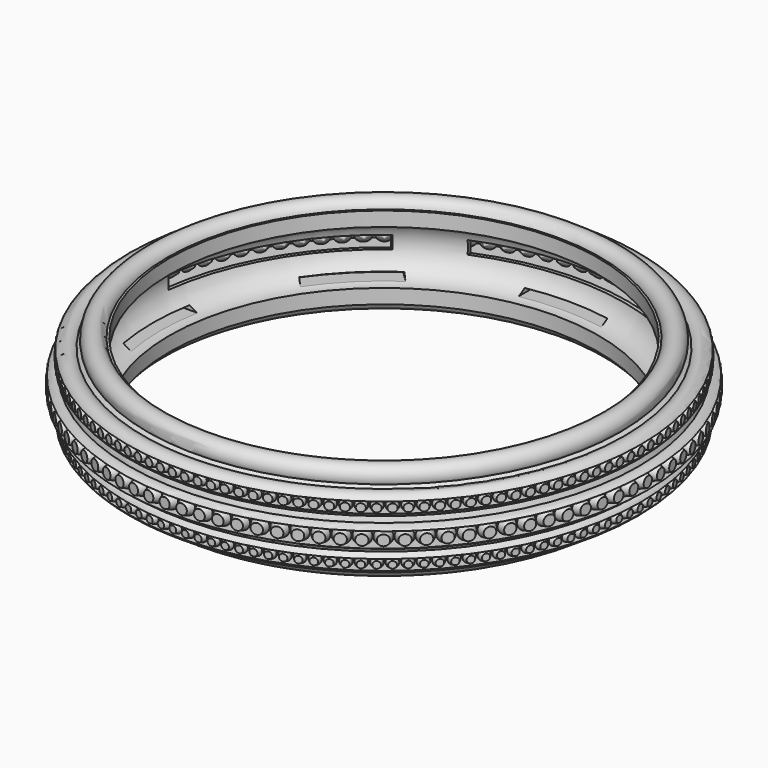
from build123d import *

# Parameters (mm, degrees)
F2_W      = 10.7606031051
F2_H      = 7.2111079935
F4_W      = 88.9
F4_H      = 6.096
F5_DEPTH  = 124.6271398151
F6_COUNT  = 6
F9_COUNT  = 98
F10_W     = 10.6947466134
F10_H     = 5.08
F10_W_2   = 9.758957445
F13_W     = 40.2778751929
F13_H     = 2.032
F13_W_2   = 39.1175959745
F14_DEPTH = 127
F15_COUNT = 8
F18_COUNT = 130
F21_COUNT = 130


with BuildPart() as f1:
    # F0 (on Front) → F1 (revolve)
    with BuildSketch(Plane.XZ):
        with BuildLine():
            ThreePointArc((101.6, 12.7), (114.3, 0), (101.6, -12.7))
            Line((101.6, -12.7), (101.6, -19.5476406297))
            ThreePointArc((101.6, -19.5476406297), (102.0112979939, -19.5433131313), (102.4224138798, -19.5303325521))
            ThreePointArc((102.4224138798, -19.5303325521), (108.4539940671, -23.3155491771), (111.4776025264, -16.8684090096))
            ThreePointArc((111.4776025264, -16.8684090096), (112.6214083664, -16.1443120574), (113.712355318, -15.3427866712))
            ThreePointArc((113.712355318, -15.3427866712), (121.1960862403, -14.7794979456), (119.6808746024, -7.4291471785))
            ThreePointArc((119.6808746024, -7.4291471785), (120.1341217826, -6.2126149032), (120.5056200226, -4.9686804834))
            ThreePointArc((120.5056200226, -4.9686804834), (126.157628275, 0), (120.5056200226, 4.9686804834))
            ThreePointArc((120.5056200226, 4.9686804834), (120.141776973, 6.1897302745), (119.6991616614, 7.3844838236))
            ThreePointArc((119.6991616614, 7.3844838236), (121.234298908, 14.8083181925), (113.674437882, 15.3726446658))
            ThreePointArc((113.674437882, 15.3726446658), (112.8348855677, 15.996487129), (111.963166428, 16.5745297301))
            ThreePointArc((111.963166428, 16.5745297301), (108.9586357212, 23.360226878), (102.6073888593, 19.5216654482))
            ThreePointArc((102.6073888593, 19.5216654482), (102.1038618421, 19.5411457553), (101.6, 19.5476406297))
            Line((101.6, 19.5476406297), (101.6, 12.7))
        make_face()
    revolve(axis=Axis((0, 0, 0.8939662948), (0, 0, -1)))

    # F2 (on Front) → F3 (revolve, cut)
    with BuildSketch(Plane.XZ):
        with Locations((121.0180819035, 0)):
            Rectangle(F2_W, F2_H)
    revolve(axis=Axis((0, 0, 0.6015782217), (0, 0, -1)), mode=Mode.SUBTRACT)

    # F4 (on Front) → F5 (cut, through all)
    with BuildSketch(Plane.XZ):
        Rectangle(F4_W, F4_H)
    f5 = extrude(amount=F5_DEPTH, mode=Mode.SUBTRACT)

    # F6: F5 ×6 about axis
    f6_axis = Axis((0, 0, 0.6015782217), (0, 0, -1))
    for i in range(1, F6_COUNT):
        add(f5.rotate(f6_axis, i * 360 / F6_COUNT), mode=Mode.SUBTRACT)

    # F10 (on Front) → F12 (revolve, cut)
    with BuildSketch(Plane.XZ):
        with Locations((118.0006936193, 11.8413660675)):
            Rectangle(F10_W, F10_H)
        with Locations((118.0006936193, -12.040737085)):
            Rectangle(F10_W_2, F10_H)
    revolve(axis=Axis((0, 0, 3.7605240941), (0, 0, -1)), mode=Mode.SUBTRACT)

    # F13 (on Front) → F14 (cut)
    with BuildSketch(Plane.XZ):
        with Locations((0, 10.9197665006)):
            Rectangle(F13_W, F13_H)
        with Locations((0, -10.9790544957)):
            Rectangle(F13_W_2, F13_H)
    f14 = extrude(amount=F14_DEPTH, mode=Mode.SUBTRACT)

    # F15: F14 ×8 about axis
    f15_axis = Axis((0, 0, 3.7605240941), (0, 0, -1))
    for i in range(1, F15_COUNT):
        add(f14.rotate(f15_axis, i * 360 / F15_COUNT), mode=Mode.SUBTRACT)


with BuildPart() as f8:
    # F7 (on Front) → F8 (revolve)
    with BuildSketch(Plane.XZ):
        Polygon((121.5662360191, 3.7640826777), (117.0876398683, 0), (124.899148941, 0), (124.899148941, 2.4697111055), align=None)
    revolve(axis=Axis((124.899148941, 0, 0), (1, 0, 0)))


with BuildPart() as f9_1:
    # F9: instance of F8
    add(f8.part.rotate(Axis((0, 0, 0.6015782217), (0, 0, -1)), 1 * 360 / F9_COUNT))


with BuildPart() as f9_2:
    # F9: instance of F8
    add(f8.part.rotate(Axis((0, 0, 0.6015782217), (0, 0, -1)), 2 * 360 / F9_COUNT))


with BuildPart() as f9_3:
    # F9: instance of F8
    add(f8.part.rotate(Axis((0, 0, 0.6015782217), (0, 0, -1)), 3 * 360 / F9_COUNT))


with BuildPart() as f9_4:
    # F9: instance of F8
    add(f8.part.rotate(Axis((0, 0, 0.6015782217), (0, 0, -1)), 4 * 360 / F9_COUNT))


with BuildPart() as f9_5:
    # F9: instance of F8
    add(f8.part.rotate(Axis((0, 0, 0.6015782217), (0, 0, -1)), 5 * 360 / F9_COUNT))


with BuildPart() as f9_6:
    # F9: instance of F8
    add(f8.part.rotate(Axis((0, 0, 0.6015782217), (0, 0, -1)), 6 * 360 / F9_COUNT))


with BuildPart() as f9_7:
    # F9: instance of F8
    add(f8.part.rotate(Axis((0, 0, 0.6015782217), (0, 0, -1)), 7 * 360 / F9_COUNT))


with BuildPart() as f9_8:
    # F9: instance of F8
    add(f8.part.rotate(Axis((0, 0, 0.6015782217), (0, 0, -1)), 8 * 360 / F9_COUNT))


with BuildPart() as f9_9:
    # F9: instance of F8
    add(f8.part.rotate(Axis((0, 0, 0.6015782217), (0, 0, -1)), 9 * 360 / F9_COUNT))


with BuildPart() as f9_10:
    # F9: instance of F8
    add(f8.part.rotate(Axis((0, 0, 0.6015782217), (0, 0, -1)), 10 * 360 / F9_COUNT))


with BuildPart() as f9_11:
    # F9: instance of F8
    add(f8.part.rotate(Axis((0, 0, 0.6015782217), (0, 0, -1)), 11 * 360 / F9_COUNT))


with BuildPart() as f9_12:
    # F9: instance of F8
    add(f8.part.rotate(Axis((0, 0, 0.6015782217), (0, 0, -1)), 12 * 360 / F9_COUNT))


with BuildPart() as f9_13:
    # F9: instance of F8
    add(f8.part.rotate(Axis((0, 0, 0.6015782217), (0, 0, -1)), 13 * 360 / F9_COUNT))


with BuildPart() as f9_14:
    # F9: instance of F8
    add(f8.part.rotate(Axis((0, 0, 0.6015782217), (0, 0, -1)), 14 * 360 / F9_COUNT))


with BuildPart() as f9_15:
    # F9: instance of F8
    add(f8.part.rotate(Axis((0, 0, 0.6015782217), (0, 0, -1)), 15 * 360 / F9_COUNT))


with BuildPart() as f9_16:
    # F9: instance of F8
    add(f8.part.rotate(Axis((0, 0, 0.6015782217), (0, 0, -1)), 16 * 360 / F9_COUNT))


with BuildPart() as f9_17:
    # F9: instance of F8
    add(f8.part.rotate(Axis((0, 0, 0.6015782217), (0, 0, -1)), 17 * 360 / F9_COUNT))


with BuildPart() as f9_18:
    # F9: instance of F8
    add(f8.part.rotate(Axis((0, 0, 0.6015782217), (0, 0, -1)), 18 * 360 / F9_COUNT))


with BuildPart() as f9_19:
    # F9: instance of F8
    add(f8.part.rotate(Axis((0, 0, 0.6015782217), (0, 0, -1)), 19 * 360 / F9_COUNT))


with BuildPart() as f9_20:
    # F9: instance of F8
    add(f8.part.rotate(Axis((0, 0, 0.6015782217), (0, 0, -1)), 20 * 360 / F9_COUNT))


with BuildPart() as f9_21:
    # F9: instance of F8
    add(f8.part.rotate(Axis((0, 0, 0.6015782217), (0, 0, -1)), 21 * 360 / F9_COUNT))


with BuildPart() as f9_22:
    # F9: instance of F8
    add(f8.part.rotate(Axis((0, 0, 0.6015782217), (0, 0, -1)), 22 * 360 / F9_COUNT))


with BuildPart() as f9_23:
    # F9: instance of F8
    add(f8.part.rotate(Axis((0, 0, 0.6015782217), (0, 0, -1)), 23 * 360 / F9_COUNT))


with BuildPart() as f9_24:
    # F9: instance of F8
    add(f8.part.rotate(Axis((0, 0, 0.6015782217), (0, 0, -1)), 24 * 360 / F9_COUNT))


with BuildPart() as f9_25:
    # F9: instance of F8
    add(f8.part.rotate(Axis((0, 0, 0.6015782217), (0, 0, -1)), 25 * 360 / F9_COUNT))


with BuildPart() as f9_26:
    # F9: instance of F8
    add(f8.part.rotate(Axis((0, 0, 0.6015782217), (0, 0, -1)), 26 * 360 / F9_COUNT))


with BuildPart() as f9_27:
    # F9: instance of F8
    add(f8.part.rotate(Axis((0, 0, 0.6015782217), (0, 0, -1)), 27 * 360 / F9_COUNT))


with BuildPart() as f9_28:
    # F9: instance of F8
    add(f8.part.rotate(Axis((0, 0, 0.6015782217), (0, 0, -1)), 28 * 360 / F9_COUNT))


with BuildPart() as f9_29:
    # F9: instance of F8
    add(f8.part.rotate(Axis((0, 0, 0.6015782217), (0, 0, -1)), 29 * 360 / F9_COUNT))


with BuildPart() as f9_30:
    # F9: instance of F8
    add(f8.part.rotate(Axis((0, 0, 0.6015782217), (0, 0, -1)), 30 * 360 / F9_COUNT))


with BuildPart() as f9_31:
    # F9: instance of F8
    add(f8.part.rotate(Axis((0, 0, 0.6015782217), (0, 0, -1)), 31 * 360 / F9_COUNT))


with BuildPart() as f9_32:
    # F9: instance of F8
    add(f8.part.rotate(Axis((0, 0, 0.6015782217), (0, 0, -1)), 32 * 360 / F9_COUNT))


with BuildPart() as f9_33:
    # F9: instance of F8
    add(f8.part.rotate(Axis((0, 0, 0.6015782217), (0, 0, -1)), 33 * 360 / F9_COUNT))


with BuildPart() as f9_34:
    # F9: instance of F8
    add(f8.part.rotate(Axis((0, 0, 0.6015782217), (0, 0, -1)), 34 * 360 / F9_COUNT))


with BuildPart() as f9_35:
    # F9: instance of F8
    add(f8.part.rotate(Axis((0, 0, 0.6015782217), (0, 0, -1)), 35 * 360 / F9_COUNT))


with BuildPart() as f9_36:
    # F9: instance of F8
    add(f8.part.rotate(Axis((0, 0, 0.6015782217), (0, 0, -1)), 36 * 360 / F9_COUNT))


with BuildPart() as f9_37:
    # F9: instance of F8
    add(f8.part.rotate(Axis((0, 0, 0.6015782217), (0, 0, -1)), 37 * 360 / F9_COUNT))


with BuildPart() as f9_38:
    # F9: instance of F8
    add(f8.part.rotate(Axis((0, 0, 0.6015782217), (0, 0, -1)), 38 * 360 / F9_COUNT))


with BuildPart() as f9_39:
    # F9: instance of F8
    add(f8.part.rotate(Axis((0, 0, 0.6015782217), (0, 0, -1)), 39 * 360 / F9_COUNT))


with BuildPart() as f9_40:
    # F9: instance of F8
    add(f8.part.rotate(Axis((0, 0, 0.6015782217), (0, 0, -1)), 40 * 360 / F9_COUNT))


with BuildPart() as f9_41:
    # F9: instance of F8
    add(f8.part.rotate(Axis((0, 0, 0.6015782217), (0, 0, -1)), 41 * 360 / F9_COUNT))


with BuildPart() as f9_42:
    # F9: instance of F8
    add(f8.part.rotate(Axis((0, 0, 0.6015782217), (0, 0, -1)), 42 * 360 / F9_COUNT))


with BuildPart() as f9_43:
    # F9: instance of F8
    add(f8.part.rotate(Axis((0, 0, 0.6015782217), (0, 0, -1)), 43 * 360 / F9_COUNT))


with BuildPart() as f9_44:
    # F9: instance of F8
    add(f8.part.rotate(Axis((0, 0, 0.6015782217), (0, 0, -1)), 44 * 360 / F9_COUNT))


with BuildPart() as f9_45:
    # F9: instance of F8
    add(f8.part.rotate(Axis((0, 0, 0.6015782217), (0, 0, -1)), 45 * 360 / F9_COUNT))


with BuildPart() as f9_46:
    # F9: instance of F8
    add(f8.part.rotate(Axis((0, 0, 0.6015782217), (0, 0, -1)), 46 * 360 / F9_COUNT))


with BuildPart() as f9_47:
    # F9: instance of F8
    add(f8.part.rotate(Axis((0, 0, 0.6015782217), (0, 0, -1)), 47 * 360 / F9_COUNT))


with BuildPart() as f9_48:
    # F9: instance of F8
    add(f8.part.rotate(Axis((0, 0, 0.6015782217), (0, 0, -1)), 48 * 360 / F9_COUNT))


with BuildPart() as f9_49:
    # F9: instance of F8
    add(f8.part.rotate(Axis((0, 0, 0.6015782217), (0, 0, -1)), 49 * 360 / F9_COUNT))


with BuildPart() as f9_50:
    # F9: instance of F8
    add(f8.part.rotate(Axis((0, 0, 0.6015782217), (0, 0, -1)), 50 * 360 / F9_COUNT))


with BuildPart() as f9_51:
    # F9: instance of F8
    add(f8.part.rotate(Axis((0, 0, 0.6015782217), (0, 0, -1)), 51 * 360 / F9_COUNT))


with BuildPart() as f9_52:
    # F9: instance of F8
    add(f8.part.rotate(Axis((0, 0, 0.6015782217), (0, 0, -1)), 52 * 360 / F9_COUNT))


with BuildPart() as f9_53:
    # F9: instance of F8
    add(f8.part.rotate(Axis((0, 0, 0.6015782217), (0, 0, -1)), 53 * 360 / F9_COUNT))


with BuildPart() as f9_54:
    # F9: instance of F8
    add(f8.part.rotate(Axis((0, 0, 0.6015782217), (0, 0, -1)), 54 * 360 / F9_COUNT))


with BuildPart() as f9_55:
    # F9: instance of F8
    add(f8.part.rotate(Axis((0, 0, 0.6015782217), (0, 0, -1)), 55 * 360 / F9_COUNT))


with BuildPart() as f9_56:
    # F9: instance of F8
    add(f8.part.rotate(Axis((0, 0, 0.6015782217), (0, 0, -1)), 56 * 360 / F9_COUNT))


with BuildPart() as f9_57:
    # F9: instance of F8
    add(f8.part.rotate(Axis((0, 0, 0.6015782217), (0, 0, -1)), 57 * 360 / F9_COUNT))


with BuildPart() as f9_58:
    # F9: instance of F8
    add(f8.part.rotate(Axis((0, 0, 0.6015782217), (0, 0, -1)), 58 * 360 / F9_COUNT))


with BuildPart() as f9_59:
    # F9: instance of F8
    add(f8.part.rotate(Axis((0, 0, 0.6015782217), (0, 0, -1)), 59 * 360 / F9_COUNT))


with BuildPart() as f9_60:
    # F9: instance of F8
    add(f8.part.rotate(Axis((0, 0, 0.6015782217), (0, 0, -1)), 60 * 360 / F9_COUNT))


with BuildPart() as f9_61:
    # F9: instance of F8
    add(f8.part.rotate(Axis((0, 0, 0.6015782217), (0, 0, -1)), 61 * 360 / F9_COUNT))


with BuildPart() as f9_62:
    # F9: instance of F8
    add(f8.part.rotate(Axis((0, 0, 0.6015782217), (0, 0, -1)), 62 * 360 / F9_COUNT))


with BuildPart() as f9_63:
    # F9: instance of F8
    add(f8.part.rotate(Axis((0, 0, 0.6015782217), (0, 0, -1)), 63 * 360 / F9_COUNT))


with BuildPart() as f9_64:
    # F9: instance of F8
    add(f8.part.rotate(Axis((0, 0, 0.6015782217), (0, 0, -1)), 64 * 360 / F9_COUNT))


with BuildPart() as f9_65:
    # F9: instance of F8
    add(f8.part.rotate(Axis((0, 0, 0.6015782217), (0, 0, -1)), 65 * 360 / F9_COUNT))


with BuildPart() as f9_66:
    # F9: instance of F8
    add(f8.part.rotate(Axis((0, 0, 0.6015782217), (0, 0, -1)), 66 * 360 / F9_COUNT))


with BuildPart() as f9_67:
    # F9: instance of F8
    add(f8.part.rotate(Axis((0, 0, 0.6015782217), (0, 0, -1)), 67 * 360 / F9_COUNT))


with BuildPart() as f9_68:
    # F9: instance of F8
    add(f8.part.rotate(Axis((0, 0, 0.6015782217), (0, 0, -1)), 68 * 360 / F9_COUNT))


with BuildPart() as f9_69:
    # F9: instance of F8
    add(f8.part.rotate(Axis((0, 0, 0.6015782217), (0, 0, -1)), 69 * 360 / F9_COUNT))


with BuildPart() as f9_70:
    # F9: instance of F8
    add(f8.part.rotate(Axis((0, 0, 0.6015782217), (0, 0, -1)), 70 * 360 / F9_COUNT))


with BuildPart() as f9_71:
    # F9: instance of F8
    add(f8.part.rotate(Axis((0, 0, 0.6015782217), (0, 0, -1)), 71 * 360 / F9_COUNT))


with BuildPart() as f9_72:
    # F9: instance of F8
    add(f8.part.rotate(Axis((0, 0, 0.6015782217), (0, 0, -1)), 72 * 360 / F9_COUNT))


with BuildPart() as f9_73:
    # F9: instance of F8
    add(f8.part.rotate(Axis((0, 0, 0.6015782217), (0, 0, -1)), 73 * 360 / F9_COUNT))


with BuildPart() as f9_74:
    # F9: instance of F8
    add(f8.part.rotate(Axis((0, 0, 0.6015782217), (0, 0, -1)), 74 * 360 / F9_COUNT))


with BuildPart() as f9_75:
    # F9: instance of F8
    add(f8.part.rotate(Axis((0, 0, 0.6015782217), (0, 0, -1)), 75 * 360 / F9_COUNT))


with BuildPart() as f9_76:
    # F9: instance of F8
    add(f8.part.rotate(Axis((0, 0, 0.6015782217), (0, 0, -1)), 76 * 360 / F9_COUNT))


with BuildPart() as f9_77:
    # F9: instance of F8
    add(f8.part.rotate(Axis((0, 0, 0.6015782217), (0, 0, -1)), 77 * 360 / F9_COUNT))


with BuildPart() as f9_78:
    # F9: instance of F8
    add(f8.part.rotate(Axis((0, 0, 0.6015782217), (0, 0, -1)), 78 * 360 / F9_COUNT))


with BuildPart() as f9_79:
    # F9: instance of F8
    add(f8.part.rotate(Axis((0, 0, 0.6015782217), (0, 0, -1)), 79 * 360 / F9_COUNT))


with BuildPart() as f9_80:
    # F9: instance of F8
    add(f8.part.rotate(Axis((0, 0, 0.6015782217), (0, 0, -1)), 80 * 360 / F9_COUNT))


with BuildPart() as f9_81:
    # F9: instance of F8
    add(f8.part.rotate(Axis((0, 0, 0.6015782217), (0, 0, -1)), 81 * 360 / F9_COUNT))


with BuildPart() as f9_82:
    # F9: instance of F8
    add(f8.part.rotate(Axis((0, 0, 0.6015782217), (0, 0, -1)), 82 * 360 / F9_COUNT))


with BuildPart() as f9_83:
    # F9: instance of F8
    add(f8.part.rotate(Axis((0, 0, 0.6015782217), (0, 0, -1)), 83 * 360 / F9_COUNT))


with BuildPart() as f9_84:
    # F9: instance of F8
    add(f8.part.rotate(Axis((0, 0, 0.6015782217), (0, 0, -1)), 84 * 360 / F9_COUNT))


with BuildPart() as f9_85:
    # F9: instance of F8
    add(f8.part.rotate(Axis((0, 0, 0.6015782217), (0, 0, -1)), 85 * 360 / F9_COUNT))


with BuildPart() as f9_86:
    # F9: instance of F8
    add(f8.part.rotate(Axis((0, 0, 0.6015782217), (0, 0, -1)), 86 * 360 / F9_COUNT))


with BuildPart() as f9_87:
    # F9: instance of F8
    add(f8.part.rotate(Axis((0, 0, 0.6015782217), (0, 0, -1)), 87 * 360 / F9_COUNT))


with BuildPart() as f9_88:
    # F9: instance of F8
    add(f8.part.rotate(Axis((0, 0, 0.6015782217), (0, 0, -1)), 88 * 360 / F9_COUNT))


with BuildPart() as f9_89:
    # F9: instance of F8
    add(f8.part.rotate(Axis((0, 0, 0.6015782217), (0, 0, -1)), 89 * 360 / F9_COUNT))


with BuildPart() as f9_90:
    # F9: instance of F8
    add(f8.part.rotate(Axis((0, 0, 0.6015782217), (0, 0, -1)), 90 * 360 / F9_COUNT))


with BuildPart() as f9_91:
    # F9: instance of F8
    add(f8.part.rotate(Axis((0, 0, 0.6015782217), (0, 0, -1)), 91 * 360 / F9_COUNT))


with BuildPart() as f9_92:
    # F9: instance of F8
    add(f8.part.rotate(Axis((0, 0, 0.6015782217), (0, 0, -1)), 92 * 360 / F9_COUNT))


with BuildPart() as f9_93:
    # F9: instance of F8
    add(f8.part.rotate(Axis((0, 0, 0.6015782217), (0, 0, -1)), 93 * 360 / F9_COUNT))


with BuildPart() as f9_94:
    # F9: instance of F8
    add(f8.part.rotate(Axis((0, 0, 0.6015782217), (0, 0, -1)), 94 * 360 / F9_COUNT))


with BuildPart() as f9_95:
    # F9: instance of F8
    add(f8.part.rotate(Axis((0, 0, 0.6015782217), (0, 0, -1)), 95 * 360 / F9_COUNT))


with BuildPart() as f9_96:
    # F9: instance of F8
    add(f8.part.rotate(Axis((0, 0, 0.6015782217), (0, 0, -1)), 96 * 360 / F9_COUNT))


with BuildPart() as f9_97:
    # F9: instance of F8
    add(f8.part.rotate(Axis((0, 0, 0.6015782217), (0, 0, -1)), 97 * 360 / F9_COUNT))


with BuildPart() as f17:
    # F16 (on Front) → F17 (revolve)
    with BuildSketch(Plane.XZ):
        Polygon((115.7522408575, 11.8132652715), (121.7399388552, 11.8132652715), (121.7399388552, 13.6975445746), (119.4161549211, 14.4187174737), align=None)
    revolve(axis=Axis((116.3177825511, 0, 11.8132652715), (1, 0, 0)))


with BuildPart() as f18_1:
    # F18: instance of F17
    add(f17.part.rotate(Axis((0, 0, 3.7605240941), (0, 0, -1)), 1 * 360 / F18_COUNT))


with BuildPart() as f18_2:
    # F18: instance of F17
    add(f17.part.rotate(Axis((0, 0, 3.7605240941), (0, 0, -1)), 2 * 360 / F18_COUNT))


with BuildPart() as f18_3:
    # F18: instance of F17
    add(f17.part.rotate(Axis((0, 0, 3.7605240941), (0, 0, -1)), 3 * 360 / F18_COUNT))


with BuildPart() as f18_4:
    # F18: instance of F17
    add(f17.part.rotate(Axis((0, 0, 3.7605240941), (0, 0, -1)), 4 * 360 / F18_COUNT))


with BuildPart() as f18_5:
    # F18: instance of F17
    add(f17.part.rotate(Axis((0, 0, 3.7605240941), (0, 0, -1)), 5 * 360 / F18_COUNT))


with BuildPart() as f18_6:
    # F18: instance of F17
    add(f17.part.rotate(Axis((0, 0, 3.7605240941), (0, 0, -1)), 6 * 360 / F18_COUNT))


with BuildPart() as f18_7:
    # F18: instance of F17
    add(f17.part.rotate(Axis((0, 0, 3.7605240941), (0, 0, -1)), 7 * 360 / F18_COUNT))


with BuildPart() as f18_8:
    # F18: instance of F17
    add(f17.part.rotate(Axis((0, 0, 3.7605240941), (0, 0, -1)), 8 * 360 / F18_COUNT))


with BuildPart() as f18_9:
    # F18: instance of F17
    add(f17.part.rotate(Axis((0, 0, 3.7605240941), (0, 0, -1)), 9 * 360 / F18_COUNT))


with BuildPart() as f18_10:
    # F18: instance of F17
    add(f17.part.rotate(Axis((0, 0, 3.7605240941), (0, 0, -1)), 10 * 360 / F18_COUNT))


with BuildPart() as f18_11:
    # F18: instance of F17
    add(f17.part.rotate(Axis((0, 0, 3.7605240941), (0, 0, -1)), 11 * 360 / F18_COUNT))


with BuildPart() as f18_12:
    # F18: instance of F17
    add(f17.part.rotate(Axis((0, 0, 3.7605240941), (0, 0, -1)), 12 * 360 / F18_COUNT))


with BuildPart() as f18_13:
    # F18: instance of F17
    add(f17.part.rotate(Axis((0, 0, 3.7605240941), (0, 0, -1)), 13 * 360 / F18_COUNT))


with BuildPart() as f18_14:
    # F18: instance of F17
    add(f17.part.rotate(Axis((0, 0, 3.7605240941), (0, 0, -1)), 14 * 360 / F18_COUNT))


with BuildPart() as f18_15:
    # F18: instance of F17
    add(f17.part.rotate(Axis((0, 0, 3.7605240941), (0, 0, -1)), 15 * 360 / F18_COUNT))


with BuildPart() as f18_16:
    # F18: instance of F17
    add(f17.part.rotate(Axis((0, 0, 3.7605240941), (0, 0, -1)), 16 * 360 / F18_COUNT))


with BuildPart() as f18_17:
    # F18: instance of F17
    add(f17.part.rotate(Axis((0, 0, 3.7605240941), (0, 0, -1)), 17 * 360 / F18_COUNT))


with BuildPart() as f18_18:
    # F18: instance of F17
    add(f17.part.rotate(Axis((0, 0, 3.7605240941), (0, 0, -1)), 18 * 360 / F18_COUNT))


with BuildPart() as f18_19:
    # F18: instance of F17
    add(f17.part.rotate(Axis((0, 0, 3.7605240941), (0, 0, -1)), 19 * 360 / F18_COUNT))


with BuildPart() as f18_20:
    # F18: instance of F17
    add(f17.part.rotate(Axis((0, 0, 3.7605240941), (0, 0, -1)), 20 * 360 / F18_COUNT))


with BuildPart() as f18_21:
    # F18: instance of F17
    add(f17.part.rotate(Axis((0, 0, 3.7605240941), (0, 0, -1)), 21 * 360 / F18_COUNT))


with BuildPart() as f18_22:
    # F18: instance of F17
    add(f17.part.rotate(Axis((0, 0, 3.7605240941), (0, 0, -1)), 22 * 360 / F18_COUNT))


with BuildPart() as f18_23:
    # F18: instance of F17
    add(f17.part.rotate(Axis((0, 0, 3.7605240941), (0, 0, -1)), 23 * 360 / F18_COUNT))


with BuildPart() as f18_24:
    # F18: instance of F17
    add(f17.part.rotate(Axis((0, 0, 3.7605240941), (0, 0, -1)), 24 * 360 / F18_COUNT))


with BuildPart() as f18_25:
    # F18: instance of F17
    add(f17.part.rotate(Axis((0, 0, 3.7605240941), (0, 0, -1)), 25 * 360 / F18_COUNT))


with BuildPart() as f18_26:
    # F18: instance of F17
    add(f17.part.rotate(Axis((0, 0, 3.7605240941), (0, 0, -1)), 26 * 360 / F18_COUNT))


with BuildPart() as f18_27:
    # F18: instance of F17
    add(f17.part.rotate(Axis((0, 0, 3.7605240941), (0, 0, -1)), 27 * 360 / F18_COUNT))


with BuildPart() as f18_28:
    # F18: instance of F17
    add(f17.part.rotate(Axis((0, 0, 3.7605240941), (0, 0, -1)), 28 * 360 / F18_COUNT))


with BuildPart() as f18_29:
    # F18: instance of F17
    add(f17.part.rotate(Axis((0, 0, 3.7605240941), (0, 0, -1)), 29 * 360 / F18_COUNT))


with BuildPart() as f18_30:
    # F18: instance of F17
    add(f17.part.rotate(Axis((0, 0, 3.7605240941), (0, 0, -1)), 30 * 360 / F18_COUNT))


with BuildPart() as f18_31:
    # F18: instance of F17
    add(f17.part.rotate(Axis((0, 0, 3.7605240941), (0, 0, -1)), 31 * 360 / F18_COUNT))


with BuildPart() as f18_32:
    # F18: instance of F17
    add(f17.part.rotate(Axis((0, 0, 3.7605240941), (0, 0, -1)), 32 * 360 / F18_COUNT))


with BuildPart() as f18_33:
    # F18: instance of F17
    add(f17.part.rotate(Axis((0, 0, 3.7605240941), (0, 0, -1)), 33 * 360 / F18_COUNT))


with BuildPart() as f18_34:
    # F18: instance of F17
    add(f17.part.rotate(Axis((0, 0, 3.7605240941), (0, 0, -1)), 34 * 360 / F18_COUNT))


with BuildPart() as f18_35:
    # F18: instance of F17
    add(f17.part.rotate(Axis((0, 0, 3.7605240941), (0, 0, -1)), 35 * 360 / F18_COUNT))


with BuildPart() as f18_36:
    # F18: instance of F17
    add(f17.part.rotate(Axis((0, 0, 3.7605240941), (0, 0, -1)), 36 * 360 / F18_COUNT))


with BuildPart() as f18_37:
    # F18: instance of F17
    add(f17.part.rotate(Axis((0, 0, 3.7605240941), (0, 0, -1)), 37 * 360 / F18_COUNT))


with BuildPart() as f18_38:
    # F18: instance of F17
    add(f17.part.rotate(Axis((0, 0, 3.7605240941), (0, 0, -1)), 38 * 360 / F18_COUNT))


with BuildPart() as f18_39:
    # F18: instance of F17
    add(f17.part.rotate(Axis((0, 0, 3.7605240941), (0, 0, -1)), 39 * 360 / F18_COUNT))


with BuildPart() as f18_40:
    # F18: instance of F17
    add(f17.part.rotate(Axis((0, 0, 3.7605240941), (0, 0, -1)), 40 * 360 / F18_COUNT))


with BuildPart() as f18_41:
    # F18: instance of F17
    add(f17.part.rotate(Axis((0, 0, 3.7605240941), (0, 0, -1)), 41 * 360 / F18_COUNT))


with BuildPart() as f18_42:
    # F18: instance of F17
    add(f17.part.rotate(Axis((0, 0, 3.7605240941), (0, 0, -1)), 42 * 360 / F18_COUNT))


with BuildPart() as f18_43:
    # F18: instance of F17
    add(f17.part.rotate(Axis((0, 0, 3.7605240941), (0, 0, -1)), 43 * 360 / F18_COUNT))


with BuildPart() as f18_44:
    # F18: instance of F17
    add(f17.part.rotate(Axis((0, 0, 3.7605240941), (0, 0, -1)), 44 * 360 / F18_COUNT))


with BuildPart() as f18_45:
    # F18: instance of F17
    add(f17.part.rotate(Axis((0, 0, 3.7605240941), (0, 0, -1)), 45 * 360 / F18_COUNT))


with BuildPart() as f18_46:
    # F18: instance of F17
    add(f17.part.rotate(Axis((0, 0, 3.7605240941), (0, 0, -1)), 46 * 360 / F18_COUNT))


with BuildPart() as f18_47:
    # F18: instance of F17
    add(f17.part.rotate(Axis((0, 0, 3.7605240941), (0, 0, -1)), 47 * 360 / F18_COUNT))


with BuildPart() as f18_48:
    # F18: instance of F17
    add(f17.part.rotate(Axis((0, 0, 3.7605240941), (0, 0, -1)), 48 * 360 / F18_COUNT))


with BuildPart() as f18_49:
    # F18: instance of F17
    add(f17.part.rotate(Axis((0, 0, 3.7605240941), (0, 0, -1)), 49 * 360 / F18_COUNT))


with BuildPart() as f18_50:
    # F18: instance of F17
    add(f17.part.rotate(Axis((0, 0, 3.7605240941), (0, 0, -1)), 50 * 360 / F18_COUNT))


with BuildPart() as f18_51:
    # F18: instance of F17
    add(f17.part.rotate(Axis((0, 0, 3.7605240941), (0, 0, -1)), 51 * 360 / F18_COUNT))


with BuildPart() as f18_52:
    # F18: instance of F17
    add(f17.part.rotate(Axis((0, 0, 3.7605240941), (0, 0, -1)), 52 * 360 / F18_COUNT))


with BuildPart() as f18_53:
    # F18: instance of F17
    add(f17.part.rotate(Axis((0, 0, 3.7605240941), (0, 0, -1)), 53 * 360 / F18_COUNT))


with BuildPart() as f18_54:
    # F18: instance of F17
    add(f17.part.rotate(Axis((0, 0, 3.7605240941), (0, 0, -1)), 54 * 360 / F18_COUNT))


with BuildPart() as f18_55:
    # F18: instance of F17
    add(f17.part.rotate(Axis((0, 0, 3.7605240941), (0, 0, -1)), 55 * 360 / F18_COUNT))


with BuildPart() as f18_56:
    # F18: instance of F17
    add(f17.part.rotate(Axis((0, 0, 3.7605240941), (0, 0, -1)), 56 * 360 / F18_COUNT))


with BuildPart() as f18_57:
    # F18: instance of F17
    add(f17.part.rotate(Axis((0, 0, 3.7605240941), (0, 0, -1)), 57 * 360 / F18_COUNT))


with BuildPart() as f18_58:
    # F18: instance of F17
    add(f17.part.rotate(Axis((0, 0, 3.7605240941), (0, 0, -1)), 58 * 360 / F18_COUNT))


with BuildPart() as f18_59:
    # F18: instance of F17
    add(f17.part.rotate(Axis((0, 0, 3.7605240941), (0, 0, -1)), 59 * 360 / F18_COUNT))


with BuildPart() as f18_60:
    # F18: instance of F17
    add(f17.part.rotate(Axis((0, 0, 3.7605240941), (0, 0, -1)), 60 * 360 / F18_COUNT))


with BuildPart() as f18_61:
    # F18: instance of F17
    add(f17.part.rotate(Axis((0, 0, 3.7605240941), (0, 0, -1)), 61 * 360 / F18_COUNT))


with BuildPart() as f18_62:
    # F18: instance of F17
    add(f17.part.rotate(Axis((0, 0, 3.7605240941), (0, 0, -1)), 62 * 360 / F18_COUNT))


with BuildPart() as f18_63:
    # F18: instance of F17
    add(f17.part.rotate(Axis((0, 0, 3.7605240941), (0, 0, -1)), 63 * 360 / F18_COUNT))


with BuildPart() as f18_64:
    # F18: instance of F17
    add(f17.part.rotate(Axis((0, 0, 3.7605240941), (0, 0, -1)), 64 * 360 / F18_COUNT))


with BuildPart() as f18_65:
    # F18: instance of F17
    add(f17.part.rotate(Axis((0, 0, 3.7605240941), (0, 0, -1)), 65 * 360 / F18_COUNT))


with BuildPart() as f18_66:
    # F18: instance of F17
    add(f17.part.rotate(Axis((0, 0, 3.7605240941), (0, 0, -1)), 66 * 360 / F18_COUNT))


with BuildPart() as f18_67:
    # F18: instance of F17
    add(f17.part.rotate(Axis((0, 0, 3.7605240941), (0, 0, -1)), 67 * 360 / F18_COUNT))


with BuildPart() as f18_68:
    # F18: instance of F17
    add(f17.part.rotate(Axis((0, 0, 3.7605240941), (0, 0, -1)), 68 * 360 / F18_COUNT))


with BuildPart() as f18_69:
    # F18: instance of F17
    add(f17.part.rotate(Axis((0, 0, 3.7605240941), (0, 0, -1)), 69 * 360 / F18_COUNT))


with BuildPart() as f18_70:
    # F18: instance of F17
    add(f17.part.rotate(Axis((0, 0, 3.7605240941), (0, 0, -1)), 70 * 360 / F18_COUNT))


with BuildPart() as f18_71:
    # F18: instance of F17
    add(f17.part.rotate(Axis((0, 0, 3.7605240941), (0, 0, -1)), 71 * 360 / F18_COUNT))


with BuildPart() as f18_72:
    # F18: instance of F17
    add(f17.part.rotate(Axis((0, 0, 3.7605240941), (0, 0, -1)), 72 * 360 / F18_COUNT))


with BuildPart() as f18_73:
    # F18: instance of F17
    add(f17.part.rotate(Axis((0, 0, 3.7605240941), (0, 0, -1)), 73 * 360 / F18_COUNT))


with BuildPart() as f18_74:
    # F18: instance of F17
    add(f17.part.rotate(Axis((0, 0, 3.7605240941), (0, 0, -1)), 74 * 360 / F18_COUNT))


with BuildPart() as f18_75:
    # F18: instance of F17
    add(f17.part.rotate(Axis((0, 0, 3.7605240941), (0, 0, -1)), 75 * 360 / F18_COUNT))


with BuildPart() as f18_76:
    # F18: instance of F17
    add(f17.part.rotate(Axis((0, 0, 3.7605240941), (0, 0, -1)), 76 * 360 / F18_COUNT))


with BuildPart() as f18_77:
    # F18: instance of F17
    add(f17.part.rotate(Axis((0, 0, 3.7605240941), (0, 0, -1)), 77 * 360 / F18_COUNT))


with BuildPart() as f18_78:
    # F18: instance of F17
    add(f17.part.rotate(Axis((0, 0, 3.7605240941), (0, 0, -1)), 78 * 360 / F18_COUNT))


with BuildPart() as f18_79:
    # F18: instance of F17
    add(f17.part.rotate(Axis((0, 0, 3.7605240941), (0, 0, -1)), 79 * 360 / F18_COUNT))


with BuildPart() as f18_80:
    # F18: instance of F17
    add(f17.part.rotate(Axis((0, 0, 3.7605240941), (0, 0, -1)), 80 * 360 / F18_COUNT))


with BuildPart() as f18_81:
    # F18: instance of F17
    add(f17.part.rotate(Axis((0, 0, 3.7605240941), (0, 0, -1)), 81 * 360 / F18_COUNT))


with BuildPart() as f18_82:
    # F18: instance of F17
    add(f17.part.rotate(Axis((0, 0, 3.7605240941), (0, 0, -1)), 82 * 360 / F18_COUNT))


with BuildPart() as f18_83:
    # F18: instance of F17
    add(f17.part.rotate(Axis((0, 0, 3.7605240941), (0, 0, -1)), 83 * 360 / F18_COUNT))


with BuildPart() as f18_84:
    # F18: instance of F17
    add(f17.part.rotate(Axis((0, 0, 3.7605240941), (0, 0, -1)), 84 * 360 / F18_COUNT))


with BuildPart() as f18_85:
    # F18: instance of F17
    add(f17.part.rotate(Axis((0, 0, 3.7605240941), (0, 0, -1)), 85 * 360 / F18_COUNT))


with BuildPart() as f18_86:
    # F18: instance of F17
    add(f17.part.rotate(Axis((0, 0, 3.7605240941), (0, 0, -1)), 86 * 360 / F18_COUNT))


with BuildPart() as f18_87:
    # F18: instance of F17
    add(f17.part.rotate(Axis((0, 0, 3.7605240941), (0, 0, -1)), 87 * 360 / F18_COUNT))


with BuildPart() as f18_88:
    # F18: instance of F17
    add(f17.part.rotate(Axis((0, 0, 3.7605240941), (0, 0, -1)), 88 * 360 / F18_COUNT))


with BuildPart() as f18_89:
    # F18: instance of F17
    add(f17.part.rotate(Axis((0, 0, 3.7605240941), (0, 0, -1)), 89 * 360 / F18_COUNT))


with BuildPart() as f18_90:
    # F18: instance of F17
    add(f17.part.rotate(Axis((0, 0, 3.7605240941), (0, 0, -1)), 90 * 360 / F18_COUNT))


with BuildPart() as f18_91:
    # F18: instance of F17
    add(f17.part.rotate(Axis((0, 0, 3.7605240941), (0, 0, -1)), 91 * 360 / F18_COUNT))


with BuildPart() as f18_92:
    # F18: instance of F17
    add(f17.part.rotate(Axis((0, 0, 3.7605240941), (0, 0, -1)), 92 * 360 / F18_COUNT))


with BuildPart() as f18_93:
    # F18: instance of F17
    add(f17.part.rotate(Axis((0, 0, 3.7605240941), (0, 0, -1)), 93 * 360 / F18_COUNT))


with BuildPart() as f18_94:
    # F18: instance of F17
    add(f17.part.rotate(Axis((0, 0, 3.7605240941), (0, 0, -1)), 94 * 360 / F18_COUNT))


with BuildPart() as f18_95:
    # F18: instance of F17
    add(f17.part.rotate(Axis((0, 0, 3.7605240941), (0, 0, -1)), 95 * 360 / F18_COUNT))


with BuildPart() as f18_96:
    # F18: instance of F17
    add(f17.part.rotate(Axis((0, 0, 3.7605240941), (0, 0, -1)), 96 * 360 / F18_COUNT))


with BuildPart() as f18_97:
    # F18: instance of F17
    add(f17.part.rotate(Axis((0, 0, 3.7605240941), (0, 0, -1)), 97 * 360 / F18_COUNT))


with BuildPart() as f18_98:
    # F18: instance of F17
    add(f17.part.rotate(Axis((0, 0, 3.7605240941), (0, 0, -1)), 98 * 360 / F18_COUNT))


with BuildPart() as f18_99:
    # F18: instance of F17
    add(f17.part.rotate(Axis((0, 0, 3.7605240941), (0, 0, -1)), 99 * 360 / F18_COUNT))


with BuildPart() as f18_100:
    # F18: instance of F17
    add(f17.part.rotate(Axis((0, 0, 3.7605240941), (0, 0, -1)), 100 * 360 / F18_COUNT))


with BuildPart() as f18_101:
    # F18: instance of F17
    add(f17.part.rotate(Axis((0, 0, 3.7605240941), (0, 0, -1)), 101 * 360 / F18_COUNT))


with BuildPart() as f18_102:
    # F18: instance of F17
    add(f17.part.rotate(Axis((0, 0, 3.7605240941), (0, 0, -1)), 102 * 360 / F18_COUNT))


with BuildPart() as f18_103:
    # F18: instance of F17
    add(f17.part.rotate(Axis((0, 0, 3.7605240941), (0, 0, -1)), 103 * 360 / F18_COUNT))


with BuildPart() as f18_104:
    # F18: instance of F17
    add(f17.part.rotate(Axis((0, 0, 3.7605240941), (0, 0, -1)), 104 * 360 / F18_COUNT))


with BuildPart() as f18_105:
    # F18: instance of F17
    add(f17.part.rotate(Axis((0, 0, 3.7605240941), (0, 0, -1)), 105 * 360 / F18_COUNT))


with BuildPart() as f18_106:
    # F18: instance of F17
    add(f17.part.rotate(Axis((0, 0, 3.7605240941), (0, 0, -1)), 106 * 360 / F18_COUNT))


with BuildPart() as f18_107:
    # F18: instance of F17
    add(f17.part.rotate(Axis((0, 0, 3.7605240941), (0, 0, -1)), 107 * 360 / F18_COUNT))


with BuildPart() as f18_108:
    # F18: instance of F17
    add(f17.part.rotate(Axis((0, 0, 3.7605240941), (0, 0, -1)), 108 * 360 / F18_COUNT))


with BuildPart() as f18_109:
    # F18: instance of F17
    add(f17.part.rotate(Axis((0, 0, 3.7605240941), (0, 0, -1)), 109 * 360 / F18_COUNT))


with BuildPart() as f18_110:
    # F18: instance of F17
    add(f17.part.rotate(Axis((0, 0, 3.7605240941), (0, 0, -1)), 110 * 360 / F18_COUNT))


with BuildPart() as f18_111:
    # F18: instance of F17
    add(f17.part.rotate(Axis((0, 0, 3.7605240941), (0, 0, -1)), 111 * 360 / F18_COUNT))


with BuildPart() as f18_112:
    # F18: instance of F17
    add(f17.part.rotate(Axis((0, 0, 3.7605240941), (0, 0, -1)), 112 * 360 / F18_COUNT))


with BuildPart() as f18_113:
    # F18: instance of F17
    add(f17.part.rotate(Axis((0, 0, 3.7605240941), (0, 0, -1)), 113 * 360 / F18_COUNT))


with BuildPart() as f18_114:
    # F18: instance of F17
    add(f17.part.rotate(Axis((0, 0, 3.7605240941), (0, 0, -1)), 114 * 360 / F18_COUNT))


with BuildPart() as f18_115:
    # F18: instance of F17
    add(f17.part.rotate(Axis((0, 0, 3.7605240941), (0, 0, -1)), 115 * 360 / F18_COUNT))


with BuildPart() as f18_116:
    # F18: instance of F17
    add(f17.part.rotate(Axis((0, 0, 3.7605240941), (0, 0, -1)), 116 * 360 / F18_COUNT))


with BuildPart() as f18_117:
    # F18: instance of F17
    add(f17.part.rotate(Axis((0, 0, 3.7605240941), (0, 0, -1)), 117 * 360 / F18_COUNT))


with BuildPart() as f18_118:
    # F18: instance of F17
    add(f17.part.rotate(Axis((0, 0, 3.7605240941), (0, 0, -1)), 118 * 360 / F18_COUNT))


with BuildPart() as f18_119:
    # F18: instance of F17
    add(f17.part.rotate(Axis((0, 0, 3.7605240941), (0, 0, -1)), 119 * 360 / F18_COUNT))


with BuildPart() as f18_120:
    # F18: instance of F17
    add(f17.part.rotate(Axis((0, 0, 3.7605240941), (0, 0, -1)), 120 * 360 / F18_COUNT))


with BuildPart() as f18_121:
    # F18: instance of F17
    add(f17.part.rotate(Axis((0, 0, 3.7605240941), (0, 0, -1)), 121 * 360 / F18_COUNT))


with BuildPart() as f18_122:
    # F18: instance of F17
    add(f17.part.rotate(Axis((0, 0, 3.7605240941), (0, 0, -1)), 122 * 360 / F18_COUNT))


with BuildPart() as f18_123:
    # F18: instance of F17
    add(f17.part.rotate(Axis((0, 0, 3.7605240941), (0, 0, -1)), 123 * 360 / F18_COUNT))


with BuildPart() as f18_124:
    # F18: instance of F17
    add(f17.part.rotate(Axis((0, 0, 3.7605240941), (0, 0, -1)), 124 * 360 / F18_COUNT))


with BuildPart() as f18_125:
    # F18: instance of F17
    add(f17.part.rotate(Axis((0, 0, 3.7605240941), (0, 0, -1)), 125 * 360 / F18_COUNT))


with BuildPart() as f18_126:
    # F18: instance of F17
    add(f17.part.rotate(Axis((0, 0, 3.7605240941), (0, 0, -1)), 126 * 360 / F18_COUNT))


with BuildPart() as f18_127:
    # F18: instance of F17
    add(f17.part.rotate(Axis((0, 0, 3.7605240941), (0, 0, -1)), 127 * 360 / F18_COUNT))


with BuildPart() as f18_128:
    # F18: instance of F17
    add(f17.part.rotate(Axis((0, 0, 3.7605240941), (0, 0, -1)), 128 * 360 / F18_COUNT))


with BuildPart() as f18_129:
    # F18: instance of F17
    add(f17.part.rotate(Axis((0, 0, 3.7605240941), (0, 0, -1)), 129 * 360 / F18_COUNT))


with BuildPart() as f20:
    # F19 (on Front) → F20 (revolve)
    with BuildSketch(Plane.XZ):
        Polygon((119.1488653421, -9.5423925668), (115.5528128147, -12.0944315568), (121.3529035449, -12.0944315568), (121.3529035449, -10.4704070836), align=None)
    revolve(axis=Axis((117.6988482475, 0, -12.0944315568), (1, 0, 0)))


with BuildPart() as f21_1:
    # F21: instance of F20
    add(f20.part.rotate(Axis((0, 0, 3.7605240941), (0, 0, -1)), 1 * 360 / F21_COUNT))


with BuildPart() as f21_2:
    # F21: instance of F20
    add(f20.part.rotate(Axis((0, 0, 3.7605240941), (0, 0, -1)), 2 * 360 / F21_COUNT))


with BuildPart() as f21_3:
    # F21: instance of F20
    add(f20.part.rotate(Axis((0, 0, 3.7605240941), (0, 0, -1)), 3 * 360 / F21_COUNT))


with BuildPart() as f21_4:
    # F21: instance of F20
    add(f20.part.rotate(Axis((0, 0, 3.7605240941), (0, 0, -1)), 4 * 360 / F21_COUNT))


with BuildPart() as f21_5:
    # F21: instance of F20
    add(f20.part.rotate(Axis((0, 0, 3.7605240941), (0, 0, -1)), 5 * 360 / F21_COUNT))


with BuildPart() as f21_6:
    # F21: instance of F20
    add(f20.part.rotate(Axis((0, 0, 3.7605240941), (0, 0, -1)), 6 * 360 / F21_COUNT))


with BuildPart() as f21_7:
    # F21: instance of F20
    add(f20.part.rotate(Axis((0, 0, 3.7605240941), (0, 0, -1)), 7 * 360 / F21_COUNT))


with BuildPart() as f21_8:
    # F21: instance of F20
    add(f20.part.rotate(Axis((0, 0, 3.7605240941), (0, 0, -1)), 8 * 360 / F21_COUNT))


with BuildPart() as f21_9:
    # F21: instance of F20
    add(f20.part.rotate(Axis((0, 0, 3.7605240941), (0, 0, -1)), 9 * 360 / F21_COUNT))


with BuildPart() as f21_10:
    # F21: instance of F20
    add(f20.part.rotate(Axis((0, 0, 3.7605240941), (0, 0, -1)), 10 * 360 / F21_COUNT))


with BuildPart() as f21_11:
    # F21: instance of F20
    add(f20.part.rotate(Axis((0, 0, 3.7605240941), (0, 0, -1)), 11 * 360 / F21_COUNT))


with BuildPart() as f21_12:
    # F21: instance of F20
    add(f20.part.rotate(Axis((0, 0, 3.7605240941), (0, 0, -1)), 12 * 360 / F21_COUNT))


with BuildPart() as f21_13:
    # F21: instance of F20
    add(f20.part.rotate(Axis((0, 0, 3.7605240941), (0, 0, -1)), 13 * 360 / F21_COUNT))


with BuildPart() as f21_14:
    # F21: instance of F20
    add(f20.part.rotate(Axis((0, 0, 3.7605240941), (0, 0, -1)), 14 * 360 / F21_COUNT))


with BuildPart() as f21_15:
    # F21: instance of F20
    add(f20.part.rotate(Axis((0, 0, 3.7605240941), (0, 0, -1)), 15 * 360 / F21_COUNT))


with BuildPart() as f21_16:
    # F21: instance of F20
    add(f20.part.rotate(Axis((0, 0, 3.7605240941), (0, 0, -1)), 16 * 360 / F21_COUNT))


with BuildPart() as f21_17:
    # F21: instance of F20
    add(f20.part.rotate(Axis((0, 0, 3.7605240941), (0, 0, -1)), 17 * 360 / F21_COUNT))


with BuildPart() as f21_18:
    # F21: instance of F20
    add(f20.part.rotate(Axis((0, 0, 3.7605240941), (0, 0, -1)), 18 * 360 / F21_COUNT))


with BuildPart() as f21_19:
    # F21: instance of F20
    add(f20.part.rotate(Axis((0, 0, 3.7605240941), (0, 0, -1)), 19 * 360 / F21_COUNT))


with BuildPart() as f21_20:
    # F21: instance of F20
    add(f20.part.rotate(Axis((0, 0, 3.7605240941), (0, 0, -1)), 20 * 360 / F21_COUNT))


with BuildPart() as f21_21:
    # F21: instance of F20
    add(f20.part.rotate(Axis((0, 0, 3.7605240941), (0, 0, -1)), 21 * 360 / F21_COUNT))


with BuildPart() as f21_22:
    # F21: instance of F20
    add(f20.part.rotate(Axis((0, 0, 3.7605240941), (0, 0, -1)), 22 * 360 / F21_COUNT))


with BuildPart() as f21_23:
    # F21: instance of F20
    add(f20.part.rotate(Axis((0, 0, 3.7605240941), (0, 0, -1)), 23 * 360 / F21_COUNT))


with BuildPart() as f21_24:
    # F21: instance of F20
    add(f20.part.rotate(Axis((0, 0, 3.7605240941), (0, 0, -1)), 24 * 360 / F21_COUNT))


with BuildPart() as f21_25:
    # F21: instance of F20
    add(f20.part.rotate(Axis((0, 0, 3.7605240941), (0, 0, -1)), 25 * 360 / F21_COUNT))


with BuildPart() as f21_26:
    # F21: instance of F20
    add(f20.part.rotate(Axis((0, 0, 3.7605240941), (0, 0, -1)), 26 * 360 / F21_COUNT))


with BuildPart() as f21_27:
    # F21: instance of F20
    add(f20.part.rotate(Axis((0, 0, 3.7605240941), (0, 0, -1)), 27 * 360 / F21_COUNT))


with BuildPart() as f21_28:
    # F21: instance of F20
    add(f20.part.rotate(Axis((0, 0, 3.7605240941), (0, 0, -1)), 28 * 360 / F21_COUNT))


with BuildPart() as f21_29:
    # F21: instance of F20
    add(f20.part.rotate(Axis((0, 0, 3.7605240941), (0, 0, -1)), 29 * 360 / F21_COUNT))


with BuildPart() as f21_30:
    # F21: instance of F20
    add(f20.part.rotate(Axis((0, 0, 3.7605240941), (0, 0, -1)), 30 * 360 / F21_COUNT))


with BuildPart() as f21_31:
    # F21: instance of F20
    add(f20.part.rotate(Axis((0, 0, 3.7605240941), (0, 0, -1)), 31 * 360 / F21_COUNT))


with BuildPart() as f21_32:
    # F21: instance of F20
    add(f20.part.rotate(Axis((0, 0, 3.7605240941), (0, 0, -1)), 32 * 360 / F21_COUNT))


with BuildPart() as f21_33:
    # F21: instance of F20
    add(f20.part.rotate(Axis((0, 0, 3.7605240941), (0, 0, -1)), 33 * 360 / F21_COUNT))


with BuildPart() as f21_34:
    # F21: instance of F20
    add(f20.part.rotate(Axis((0, 0, 3.7605240941), (0, 0, -1)), 34 * 360 / F21_COUNT))


with BuildPart() as f21_35:
    # F21: instance of F20
    add(f20.part.rotate(Axis((0, 0, 3.7605240941), (0, 0, -1)), 35 * 360 / F21_COUNT))


with BuildPart() as f21_36:
    # F21: instance of F20
    add(f20.part.rotate(Axis((0, 0, 3.7605240941), (0, 0, -1)), 36 * 360 / F21_COUNT))


with BuildPart() as f21_37:
    # F21: instance of F20
    add(f20.part.rotate(Axis((0, 0, 3.7605240941), (0, 0, -1)), 37 * 360 / F21_COUNT))


with BuildPart() as f21_38:
    # F21: instance of F20
    add(f20.part.rotate(Axis((0, 0, 3.7605240941), (0, 0, -1)), 38 * 360 / F21_COUNT))


with BuildPart() as f21_39:
    # F21: instance of F20
    add(f20.part.rotate(Axis((0, 0, 3.7605240941), (0, 0, -1)), 39 * 360 / F21_COUNT))


with BuildPart() as f21_40:
    # F21: instance of F20
    add(f20.part.rotate(Axis((0, 0, 3.7605240941), (0, 0, -1)), 40 * 360 / F21_COUNT))


with BuildPart() as f21_41:
    # F21: instance of F20
    add(f20.part.rotate(Axis((0, 0, 3.7605240941), (0, 0, -1)), 41 * 360 / F21_COUNT))


with BuildPart() as f21_42:
    # F21: instance of F20
    add(f20.part.rotate(Axis((0, 0, 3.7605240941), (0, 0, -1)), 42 * 360 / F21_COUNT))


with BuildPart() as f21_43:
    # F21: instance of F20
    add(f20.part.rotate(Axis((0, 0, 3.7605240941), (0, 0, -1)), 43 * 360 / F21_COUNT))


with BuildPart() as f21_44:
    # F21: instance of F20
    add(f20.part.rotate(Axis((0, 0, 3.7605240941), (0, 0, -1)), 44 * 360 / F21_COUNT))


with BuildPart() as f21_45:
    # F21: instance of F20
    add(f20.part.rotate(Axis((0, 0, 3.7605240941), (0, 0, -1)), 45 * 360 / F21_COUNT))


with BuildPart() as f21_46:
    # F21: instance of F20
    add(f20.part.rotate(Axis((0, 0, 3.7605240941), (0, 0, -1)), 46 * 360 / F21_COUNT))


with BuildPart() as f21_47:
    # F21: instance of F20
    add(f20.part.rotate(Axis((0, 0, 3.7605240941), (0, 0, -1)), 47 * 360 / F21_COUNT))


with BuildPart() as f21_48:
    # F21: instance of F20
    add(f20.part.rotate(Axis((0, 0, 3.7605240941), (0, 0, -1)), 48 * 360 / F21_COUNT))


with BuildPart() as f21_49:
    # F21: instance of F20
    add(f20.part.rotate(Axis((0, 0, 3.7605240941), (0, 0, -1)), 49 * 360 / F21_COUNT))


with BuildPart() as f21_50:
    # F21: instance of F20
    add(f20.part.rotate(Axis((0, 0, 3.7605240941), (0, 0, -1)), 50 * 360 / F21_COUNT))


with BuildPart() as f21_51:
    # F21: instance of F20
    add(f20.part.rotate(Axis((0, 0, 3.7605240941), (0, 0, -1)), 51 * 360 / F21_COUNT))


with BuildPart() as f21_52:
    # F21: instance of F20
    add(f20.part.rotate(Axis((0, 0, 3.7605240941), (0, 0, -1)), 52 * 360 / F21_COUNT))


with BuildPart() as f21_53:
    # F21: instance of F20
    add(f20.part.rotate(Axis((0, 0, 3.7605240941), (0, 0, -1)), 53 * 360 / F21_COUNT))


with BuildPart() as f21_54:
    # F21: instance of F20
    add(f20.part.rotate(Axis((0, 0, 3.7605240941), (0, 0, -1)), 54 * 360 / F21_COUNT))


with BuildPart() as f21_55:
    # F21: instance of F20
    add(f20.part.rotate(Axis((0, 0, 3.7605240941), (0, 0, -1)), 55 * 360 / F21_COUNT))


with BuildPart() as f21_56:
    # F21: instance of F20
    add(f20.part.rotate(Axis((0, 0, 3.7605240941), (0, 0, -1)), 56 * 360 / F21_COUNT))


with BuildPart() as f21_57:
    # F21: instance of F20
    add(f20.part.rotate(Axis((0, 0, 3.7605240941), (0, 0, -1)), 57 * 360 / F21_COUNT))


with BuildPart() as f21_58:
    # F21: instance of F20
    add(f20.part.rotate(Axis((0, 0, 3.7605240941), (0, 0, -1)), 58 * 360 / F21_COUNT))


with BuildPart() as f21_59:
    # F21: instance of F20
    add(f20.part.rotate(Axis((0, 0, 3.7605240941), (0, 0, -1)), 59 * 360 / F21_COUNT))


with BuildPart() as f21_60:
    # F21: instance of F20
    add(f20.part.rotate(Axis((0, 0, 3.7605240941), (0, 0, -1)), 60 * 360 / F21_COUNT))


with BuildPart() as f21_61:
    # F21: instance of F20
    add(f20.part.rotate(Axis((0, 0, 3.7605240941), (0, 0, -1)), 61 * 360 / F21_COUNT))


with BuildPart() as f21_62:
    # F21: instance of F20
    add(f20.part.rotate(Axis((0, 0, 3.7605240941), (0, 0, -1)), 62 * 360 / F21_COUNT))


with BuildPart() as f21_63:
    # F21: instance of F20
    add(f20.part.rotate(Axis((0, 0, 3.7605240941), (0, 0, -1)), 63 * 360 / F21_COUNT))


with BuildPart() as f21_64:
    # F21: instance of F20
    add(f20.part.rotate(Axis((0, 0, 3.7605240941), (0, 0, -1)), 64 * 360 / F21_COUNT))


with BuildPart() as f21_65:
    # F21: instance of F20
    add(f20.part.rotate(Axis((0, 0, 3.7605240941), (0, 0, -1)), 65 * 360 / F21_COUNT))


with BuildPart() as f21_66:
    # F21: instance of F20
    add(f20.part.rotate(Axis((0, 0, 3.7605240941), (0, 0, -1)), 66 * 360 / F21_COUNT))


with BuildPart() as f21_67:
    # F21: instance of F20
    add(f20.part.rotate(Axis((0, 0, 3.7605240941), (0, 0, -1)), 67 * 360 / F21_COUNT))


with BuildPart() as f21_68:
    # F21: instance of F20
    add(f20.part.rotate(Axis((0, 0, 3.7605240941), (0, 0, -1)), 68 * 360 / F21_COUNT))


with BuildPart() as f21_69:
    # F21: instance of F20
    add(f20.part.rotate(Axis((0, 0, 3.7605240941), (0, 0, -1)), 69 * 360 / F21_COUNT))


with BuildPart() as f21_70:
    # F21: instance of F20
    add(f20.part.rotate(Axis((0, 0, 3.7605240941), (0, 0, -1)), 70 * 360 / F21_COUNT))


with BuildPart() as f21_71:
    # F21: instance of F20
    add(f20.part.rotate(Axis((0, 0, 3.7605240941), (0, 0, -1)), 71 * 360 / F21_COUNT))


with BuildPart() as f21_72:
    # F21: instance of F20
    add(f20.part.rotate(Axis((0, 0, 3.7605240941), (0, 0, -1)), 72 * 360 / F21_COUNT))


with BuildPart() as f21_73:
    # F21: instance of F20
    add(f20.part.rotate(Axis((0, 0, 3.7605240941), (0, 0, -1)), 73 * 360 / F21_COUNT))


with BuildPart() as f21_74:
    # F21: instance of F20
    add(f20.part.rotate(Axis((0, 0, 3.7605240941), (0, 0, -1)), 74 * 360 / F21_COUNT))


with BuildPart() as f21_75:
    # F21: instance of F20
    add(f20.part.rotate(Axis((0, 0, 3.7605240941), (0, 0, -1)), 75 * 360 / F21_COUNT))


with BuildPart() as f21_76:
    # F21: instance of F20
    add(f20.part.rotate(Axis((0, 0, 3.7605240941), (0, 0, -1)), 76 * 360 / F21_COUNT))


with BuildPart() as f21_77:
    # F21: instance of F20
    add(f20.part.rotate(Axis((0, 0, 3.7605240941), (0, 0, -1)), 77 * 360 / F21_COUNT))


with BuildPart() as f21_78:
    # F21: instance of F20
    add(f20.part.rotate(Axis((0, 0, 3.7605240941), (0, 0, -1)), 78 * 360 / F21_COUNT))


with BuildPart() as f21_79:
    # F21: instance of F20
    add(f20.part.rotate(Axis((0, 0, 3.7605240941), (0, 0, -1)), 79 * 360 / F21_COUNT))


with BuildPart() as f21_80:
    # F21: instance of F20
    add(f20.part.rotate(Axis((0, 0, 3.7605240941), (0, 0, -1)), 80 * 360 / F21_COUNT))


with BuildPart() as f21_81:
    # F21: instance of F20
    add(f20.part.rotate(Axis((0, 0, 3.7605240941), (0, 0, -1)), 81 * 360 / F21_COUNT))


with BuildPart() as f21_82:
    # F21: instance of F20
    add(f20.part.rotate(Axis((0, 0, 3.7605240941), (0, 0, -1)), 82 * 360 / F21_COUNT))


with BuildPart() as f21_83:
    # F21: instance of F20
    add(f20.part.rotate(Axis((0, 0, 3.7605240941), (0, 0, -1)), 83 * 360 / F21_COUNT))


with BuildPart() as f21_84:
    # F21: instance of F20
    add(f20.part.rotate(Axis((0, 0, 3.7605240941), (0, 0, -1)), 84 * 360 / F21_COUNT))


with BuildPart() as f21_85:
    # F21: instance of F20
    add(f20.part.rotate(Axis((0, 0, 3.7605240941), (0, 0, -1)), 85 * 360 / F21_COUNT))


with BuildPart() as f21_86:
    # F21: instance of F20
    add(f20.part.rotate(Axis((0, 0, 3.7605240941), (0, 0, -1)), 86 * 360 / F21_COUNT))


with BuildPart() as f21_87:
    # F21: instance of F20
    add(f20.part.rotate(Axis((0, 0, 3.7605240941), (0, 0, -1)), 87 * 360 / F21_COUNT))


with BuildPart() as f21_88:
    # F21: instance of F20
    add(f20.part.rotate(Axis((0, 0, 3.7605240941), (0, 0, -1)), 88 * 360 / F21_COUNT))


with BuildPart() as f21_89:
    # F21: instance of F20
    add(f20.part.rotate(Axis((0, 0, 3.7605240941), (0, 0, -1)), 89 * 360 / F21_COUNT))


with BuildPart() as f21_90:
    # F21: instance of F20
    add(f20.part.rotate(Axis((0, 0, 3.7605240941), (0, 0, -1)), 90 * 360 / F21_COUNT))


with BuildPart() as f21_91:
    # F21: instance of F20
    add(f20.part.rotate(Axis((0, 0, 3.7605240941), (0, 0, -1)), 91 * 360 / F21_COUNT))


with BuildPart() as f21_92:
    # F21: instance of F20
    add(f20.part.rotate(Axis((0, 0, 3.7605240941), (0, 0, -1)), 92 * 360 / F21_COUNT))


with BuildPart() as f21_93:
    # F21: instance of F20
    add(f20.part.rotate(Axis((0, 0, 3.7605240941), (0, 0, -1)), 93 * 360 / F21_COUNT))


with BuildPart() as f21_94:
    # F21: instance of F20
    add(f20.part.rotate(Axis((0, 0, 3.7605240941), (0, 0, -1)), 94 * 360 / F21_COUNT))


with BuildPart() as f21_95:
    # F21: instance of F20
    add(f20.part.rotate(Axis((0, 0, 3.7605240941), (0, 0, -1)), 95 * 360 / F21_COUNT))


with BuildPart() as f21_96:
    # F21: instance of F20
    add(f20.part.rotate(Axis((0, 0, 3.7605240941), (0, 0, -1)), 96 * 360 / F21_COUNT))


with BuildPart() as f21_97:
    # F21: instance of F20
    add(f20.part.rotate(Axis((0, 0, 3.7605240941), (0, 0, -1)), 97 * 360 / F21_COUNT))


with BuildPart() as f21_98:
    # F21: instance of F20
    add(f20.part.rotate(Axis((0, 0, 3.7605240941), (0, 0, -1)), 98 * 360 / F21_COUNT))


with BuildPart() as f21_99:
    # F21: instance of F20
    add(f20.part.rotate(Axis((0, 0, 3.7605240941), (0, 0, -1)), 99 * 360 / F21_COUNT))


with BuildPart() as f21_100:
    # F21: instance of F20
    add(f20.part.rotate(Axis((0, 0, 3.7605240941), (0, 0, -1)), 100 * 360 / F21_COUNT))


with BuildPart() as f21_101:
    # F21: instance of F20
    add(f20.part.rotate(Axis((0, 0, 3.7605240941), (0, 0, -1)), 101 * 360 / F21_COUNT))


with BuildPart() as f21_102:
    # F21: instance of F20
    add(f20.part.rotate(Axis((0, 0, 3.7605240941), (0, 0, -1)), 102 * 360 / F21_COUNT))


with BuildPart() as f21_103:
    # F21: instance of F20
    add(f20.part.rotate(Axis((0, 0, 3.7605240941), (0, 0, -1)), 103 * 360 / F21_COUNT))


with BuildPart() as f21_104:
    # F21: instance of F20
    add(f20.part.rotate(Axis((0, 0, 3.7605240941), (0, 0, -1)), 104 * 360 / F21_COUNT))


with BuildPart() as f21_105:
    # F21: instance of F20
    add(f20.part.rotate(Axis((0, 0, 3.7605240941), (0, 0, -1)), 105 * 360 / F21_COUNT))


with BuildPart() as f21_106:
    # F21: instance of F20
    add(f20.part.rotate(Axis((0, 0, 3.7605240941), (0, 0, -1)), 106 * 360 / F21_COUNT))


with BuildPart() as f21_107:
    # F21: instance of F20
    add(f20.part.rotate(Axis((0, 0, 3.7605240941), (0, 0, -1)), 107 * 360 / F21_COUNT))


with BuildPart() as f21_108:
    # F21: instance of F20
    add(f20.part.rotate(Axis((0, 0, 3.7605240941), (0, 0, -1)), 108 * 360 / F21_COUNT))


with BuildPart() as f21_109:
    # F21: instance of F20
    add(f20.part.rotate(Axis((0, 0, 3.7605240941), (0, 0, -1)), 109 * 360 / F21_COUNT))


with BuildPart() as f21_110:
    # F21: instance of F20
    add(f20.part.rotate(Axis((0, 0, 3.7605240941), (0, 0, -1)), 110 * 360 / F21_COUNT))


with BuildPart() as f21_111:
    # F21: instance of F20
    add(f20.part.rotate(Axis((0, 0, 3.7605240941), (0, 0, -1)), 111 * 360 / F21_COUNT))


with BuildPart() as f21_112:
    # F21: instance of F20
    add(f20.part.rotate(Axis((0, 0, 3.7605240941), (0, 0, -1)), 112 * 360 / F21_COUNT))


with BuildPart() as f21_113:
    # F21: instance of F20
    add(f20.part.rotate(Axis((0, 0, 3.7605240941), (0, 0, -1)), 113 * 360 / F21_COUNT))


with BuildPart() as f21_114:
    # F21: instance of F20
    add(f20.part.rotate(Axis((0, 0, 3.7605240941), (0, 0, -1)), 114 * 360 / F21_COUNT))


with BuildPart() as f21_115:
    # F21: instance of F20
    add(f20.part.rotate(Axis((0, 0, 3.7605240941), (0, 0, -1)), 115 * 360 / F21_COUNT))


with BuildPart() as f21_116:
    # F21: instance of F20
    add(f20.part.rotate(Axis((0, 0, 3.7605240941), (0, 0, -1)), 116 * 360 / F21_COUNT))


with BuildPart() as f21_117:
    # F21: instance of F20
    add(f20.part.rotate(Axis((0, 0, 3.7605240941), (0, 0, -1)), 117 * 360 / F21_COUNT))


with BuildPart() as f21_118:
    # F21: instance of F20
    add(f20.part.rotate(Axis((0, 0, 3.7605240941), (0, 0, -1)), 118 * 360 / F21_COUNT))


with BuildPart() as f21_119:
    # F21: instance of F20
    add(f20.part.rotate(Axis((0, 0, 3.7605240941), (0, 0, -1)), 119 * 360 / F21_COUNT))


with BuildPart() as f21_120:
    # F21: instance of F20
    add(f20.part.rotate(Axis((0, 0, 3.7605240941), (0, 0, -1)), 120 * 360 / F21_COUNT))


with BuildPart() as f21_121:
    # F21: instance of F20
    add(f20.part.rotate(Axis((0, 0, 3.7605240941), (0, 0, -1)), 121 * 360 / F21_COUNT))


with BuildPart() as f21_122:
    # F21: instance of F20
    add(f20.part.rotate(Axis((0, 0, 3.7605240941), (0, 0, -1)), 122 * 360 / F21_COUNT))


with BuildPart() as f21_123:
    # F21: instance of F20
    add(f20.part.rotate(Axis((0, 0, 3.7605240941), (0, 0, -1)), 123 * 360 / F21_COUNT))


with BuildPart() as f21_124:
    # F21: instance of F20
    add(f20.part.rotate(Axis((0, 0, 3.7605240941), (0, 0, -1)), 124 * 360 / F21_COUNT))


with BuildPart() as f21_125:
    # F21: instance of F20
    add(f20.part.rotate(Axis((0, 0, 3.7605240941), (0, 0, -1)), 125 * 360 / F21_COUNT))


with BuildPart() as f21_126:
    # F21: instance of F20
    add(f20.part.rotate(Axis((0, 0, 3.7605240941), (0, 0, -1)), 126 * 360 / F21_COUNT))


with BuildPart() as f21_127:
    # F21: instance of F20
    add(f20.part.rotate(Axis((0, 0, 3.7605240941), (0, 0, -1)), 127 * 360 / F21_COUNT))


with BuildPart() as f21_128:
    # F21: instance of F20
    add(f20.part.rotate(Axis((0, 0, 3.7605240941), (0, 0, -1)), 128 * 360 / F21_COUNT))


with BuildPart() as f21_129:
    # F21: instance of F20
    add(f20.part.rotate(Axis((0, 0, 3.7605240941), (0, 0, -1)), 129 * 360 / F21_COUNT))


solid = Compound([f1.part, f8.part, f9_1.part, f9_2.part, f9_3.part, f9_4.part, f9_5.part, f9_6.part, f9_7.part, f9_8.part, f9_9.part, f9_10.part, f9_11.part, f9_12.part, f9_13.part, f9_14.part, f9_15.part, f9_16.part, f9_17.part, f9_18.part, f9_19.part, f9_20.part, f9_21.part, f9_22.part, f9_23.part, f9_24.part, f9_25.part, f9_26.part, f9_27.part, f9_28.part, f9_29.part, f9_30.part, f9_31.part, f9_32.part, f9_33.part, f9_34.part, f9_35.part, f9_36.part, f9_37.part, f9_38.part, f9_39.part, f9_40.part, f9_41.part, f9_42.part, f9_43.part, f9_44.part, f9_45.part, f9_46.part, f9_47.part, f9_48.part, f9_49.part, f9_50.part, f9_51.part, f9_52.part, f9_53.part, f9_54.part, f9_55.part, f9_56.part, f9_57.part, f9_58.part, f9_59.part, f9_60.part, f9_61.part, f9_62.part, f9_63.part, f9_64.part, f9_65.part, f9_66.part, f9_67.part, f9_68.part, f9_69.part, f9_70.part, f9_71.part, f9_72.part, f9_73.part, f9_74.part, f9_75.part, f9_76.part, f9_77.part, f9_78.part, f9_79.part, f9_80.part, f9_81.part, f9_82.part, f9_83.part, f9_84.part, f9_85.part, f9_86.part, f9_87.part, f9_88.part, f9_89.part, f9_90.part, f9_91.part, f9_92.part, f9_93.part, f9_94.part, f9_95.part, f9_96.part, f9_97.part, f17.part, f18_1.part, f18_2.part, f18_3.part, f18_4.part, f18_5.part, f18_6.part, f18_7.part, f18_8.part, f18_9.part, f18_10.part, f18_11.part, f18_12.part, f18_13.part, f18_14.part, f18_15.part, f18_16.part, f18_17.part, f18_18.part, f18_19.part, f18_20.part, f18_21.part, f18_22.part, f18_23.part, f18_24.part, f18_25.part, f18_26.part, f18_27.part, f18_28.part, f18_29.part, f18_30.part, f18_31.part, f18_32.part, f18_33.part, f18_34.part, f18_35.part, f18_36.part, f18_37.part, f18_38.part, f18_39.part, f18_40.part, f18_41.part, f18_42.part, f18_43.part, f18_44.part, f18_45.part, f18_46.part, f18_47.part, f18_48.part, f18_49.part, f18_50.part, f18_51.part, f18_52.part, f18_53.part, f18_54.part, f18_55.part, f18_56.part, f18_57.part, f18_58.part, f18_59.part, f18_60.part, f18_61.part, f18_62.part, f18_63.part, f18_64.part, f18_65.part, f18_66.part, f18_67.part, f18_68.part, f18_69.part, f18_70.part, f18_71.part, f18_72.part, f18_73.part, f18_74.part, f18_75.part, f18_76.part, f18_77.part, f18_78.part, f18_79.part, f18_80.part, f18_81.part, f18_82.part, f18_83.part, f18_84.part, f18_85.part, f18_86.part, f18_87.part, f18_88.part, f18_89.part, f18_90.part, f18_91.part, f18_92.part, f18_93.part, f18_94.part, f18_95.part, f18_96.part, f18_97.part, f18_98.part, f18_99.part, f18_100.part, f18_101.part, f18_102.part, f18_103.part, f18_104.part, f18_105.part, f18_106.part, f18_107.part, f18_108.part, f18_109.part, f18_110.part, f18_111.part, f18_112.part, f18_113.part, f18_114.part, f18_115.part, f18_116.part, f18_117.part, f18_118.part, f18_119.part, f18_120.part, f18_121.part, f18_122.part, f18_123.part, f18_124.part, f18_125.part, f18_126.part, f18_127.part, f18_128.part, f18_129.part, f20.part, f21_1.part, f21_2.part, f21_3.part, f21_4.part, f21_5.part, f21_6.part, f21_7.part, f21_8.part, f21_9.part, f21_10.part, f21_11.part, f21_12.part, f21_13.part, f21_14.part, f21_15.part, f21_16.part, f21_17.part, f21_18.part, f21_19.part, f21_20.part, f21_21.part, f21_22.part, f21_23.part, f21_24.part, f21_25.part, f21_26.part, f21_27.part, f21_28.part, f21_29.part, f21_30.part, f21_31.part, f21_32.part, f21_33.part, f21_34.part, f21_35.part, f21_36.part, f21_37.part, f21_38.part, f21_39.part, f21_40.part, f21_41.part, f21_42.part, f21_43.part, f21_44.part, f21_45.part, f21_46.part, f21_47.part, f21_48.part, f21_49.part, f21_50.part, f21_51.part, f21_52.part, f21_53.part, f21_54.part, f21_55.part, f21_56.part, f21_57.part, f21_58.part, f21_59.part, f21_60.part, f21_61.part, f21_62.part, f21_63.part, f21_64.part, f21_65.part, f21_66.part, f21_67.part, f21_68.part, f21_69.part, f21_70.part, f21_71.part, f21_72.part, f21_73.part, f21_74.part, f21_75.part, f21_76.part, f21_77.part, f21_78.part, f21_79.part, f21_80.part, f21_81.part, f21_82.part, f21_83.part, f21_84.part, f21_85.part, f21_86.part, f21_87.part, f21_88.part, f21_89.part, f21_90.part, f21_91.part, f21_92.part, f21_93.part, f21_94.part, f21_95.part, f21_96.part, f21_97.part, f21_98.part, f21_99.part, f21_100.part, f21_101.part, f21_102.part, f21_103.part, f21_104.part, f21_105.part, f21_106.part, f21_107.part, f21_108.part, f21_109.part, f21_110.part, f21_111.part, f21_112.part, f21_113.part, f21_114.part, f21_115.part, f21_116.part, f21_117.part, f21_118.part, f21_119.part, f21_120.part, f21_121.part, f21_122.part, f21_123.part, f21_124.part, f21_125.part, f21_126.part, f21_127.part, f21_128.part, f21_129.part])
